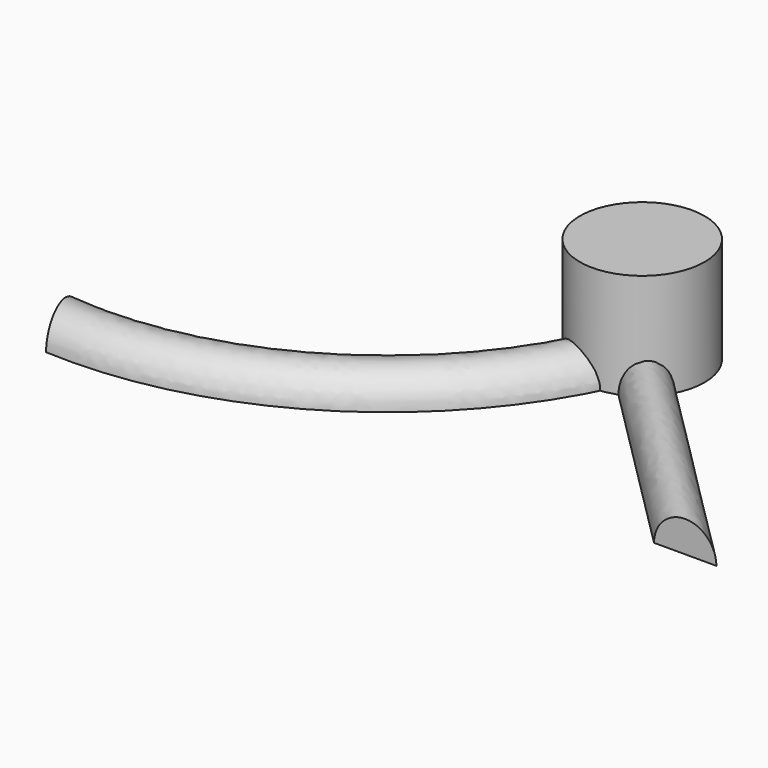
from build123d import *

# Parameters (mm, degrees)
F0_R     = 25.4
F1_DEPTH = 43.18


with BuildPart() as f1:
    # F0 (on Top) → F1 (new body)
    with BuildSketch(Plane.XY):
        Circle(F0_R)
    extrude(amount=F1_DEPTH)


with BuildPart() as f1_1:
    # F2: moved
    add(f1.part.moved(Location((0, -74.90282, 0))))


with BuildPart() as f5:
    # F5: sweep along a path in F4
    with BuildLine(Plane.XY) as f5_path:
        ThreePointArc((-154.3728560209, -100.5693227053), (-60.0449476944, -76.5966539329), (0, 0))
    # F3 (on Front) → F5 (sweep)
    with BuildSketch(Plane.XZ):
        with BuildLine():
            Line((-12.7, 0), (12.7, 0))
            ThreePointArc((12.7, 0), (0, 12.7), (-12.7, 0))
        make_face()
    sweep(path=f5_path.line)

    # F7: sweep along a path in F6
    with BuildLine(Plane.XY) as f7_path:
        Line((0, 0), (94.5657914659, -94.5657914659))
    # F5_face (on face) → F7 (sweep)
    with BuildSketch(Plane(origin=(0, 0, 5.390047406), x_dir=(-1, 0, 0), z_dir=(0, 1, 0))):
        with BuildLine():
            Line((-12.7, -5.390047406), (12.7, -5.390047406))
            ThreePointArc((12.7, -5.390047406), (0, 7.309952594), (-12.7, -5.390047406))
        make_face()
    sweep(path=f7_path.line)


with BuildPart() as f1_2:
    # F8: moved
    add(f1_1.part.moved(Location((0, 76.64604, 0))))


solid = Compound([f5.part, f1_2.part])
